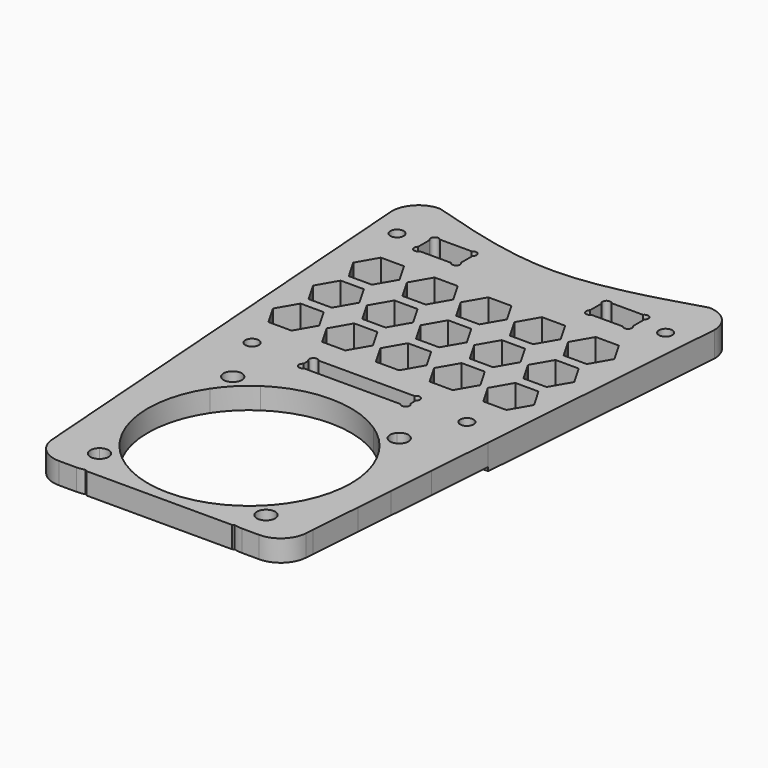
from build123d import *

# Parameters (mm, degrees)
F0_R        = 1.25
F1_DEPTH    = 4.7
F2_T1_DEPTH = 11.3905223792
F3_DEPTH    = 0.7


# Not quite as in the source:
# - a fillet or chamfer that OpenCascade refuses, or shapes differently, is made with other operations: its cross-section is extruded or revolved along the edge and cut away or added
# - a feature names something its author has since deleted; it is built from what else it names


with BuildPart() as f1:
    # F0 (on Top) → F1 (new body)
    with BuildSketch(Plane.XY):
        with BuildLine():
            ThreePointArc((-9.7202698736, -21.9205183333), (-9.7716697619, -20.7913807953), (-8.645995483, -20.8936106643))
            Line((-8.645995483, -20.8936106643), (-6.1283866754, -20.8936106643))
            Line((-6.1283866754, -20.8936106643), (-5.2063139262, -20.511675626))
            Line((-5.2063139262, -20.511675626), (0.2797301264, -20.511675626))
            Line((0.2797301264, -20.511675626), (5.7808356466, -20.511675626))
            Line((5.7808356466, -20.511675626), (6.7029083959, -20.8936106643))
            Line((6.7029083959, -20.8936106643), (9.1898135649, -20.8936106643))
            ThreePointArc((9.1898135649, -20.8936106643), (10.0314546269, -20.5883121331), (10.5658325406, -21.3066484859))
            ThreePointArc((10.5658325406, -21.3066484859), (10.4905262449, -21.6341975743), (10.2797301264, -21.8959693067))
            Line((10.2797301264, -21.8959693067), (10.2797301264, -22.3751787353))
            Line((10.2797301264, -22.3751787353), (15.9316382574, -24.7162757364))
            Line((15.9316382574, -24.7162757364), (16.8589731853, -25.6436106643))
            Line((16.8589731853, -25.6436106643), (26.7490972687, -25.6436106643))
            Line((26.7490972687, -25.6436106643), (30.2797301264, 22.5885286684))
            ThreePointArc((30.2797301264, 22.5885286684), (28.8152640324, 26.1240625744), (25.2797301264, 27.5885286684))
            add(Edge.make_bspline(
                [(-24.7202698736, 27.4813893357), (-16.3886704683, 24.9819095141), (0.2883997674, 19.9278415244), (16.944662865, 25.08800849), (25.2797301264, 27.5885286684)],
                knots=[0, 0, 0, 0, 0.4998959643, 1, 1, 1, 1], degree=3))
            ThreePointArc((-24.7202698736, 27.4813893357), (-28.2558037795, 26.0169232416), (-29.7202698736, 22.4813893357))
            Line((-29.7202698736, 22.4813893357), (-26.1974797044, -25.6436106643))
            Line((-26.1974797044, -25.6436106643), (-16.2844514649, -25.6436106643))
            Line((-16.2844514649, -25.6436106643), (-15.357116537, -24.7162757364))
            Line((-15.357116537, -24.7162757364), (-9.7202698736, -22.3814173994))
            Line((-9.7202698736, -22.3814173994), (-9.7202698736, -21.9205183333))
        make_face()
        with Locations((-19.7202698736, -22.5186106643)):
            Circle(F0_R, mode=Mode.SUBTRACT)
        Polygon((-21.9045679364, -8.5128274316), (-17.5941435837, -8.5128274316), (-15.4389314074, -12.2457644222), (-17.5941435837, -15.9787014127), (-21.9045679364, -15.9787014127), (-24.0597801128, -12.2457644222), align=None, mode=Mode.SUBTRACT)
        Polygon((-21.8574822097, 0.7808977612), (-17.547057857, 0.7808977612), (-15.3918456806, -2.9520392293), (-17.547057857, -6.6849762199), (-21.8574822097, -6.6849762199), (-24.012694386, -2.9520392293), align=None, mode=Mode.SUBTRACT)
        Polygon((-11.9045679364, -8.5128274316), (-7.5941435837, -8.5128274316), (-5.4389314074, -12.2457644222), (-7.5941435837, -15.9787014127), (-11.9045679364, -15.9787014127), (-14.0597801128, -12.2457644222), align=None, mode=Mode.SUBTRACT)
        Polygon((2.4058564163, -15.9787014127), (0.2797301264, -15.9787014127), (-1.9045679364, -15.9787014127), (-4.0597801128, -12.2457644222), (-1.9045679364, -8.5128274316), (0.2797301264, -8.5128274316), (2.4058564163, -8.5128274316), (4.5610685926, -12.2457644222), align=None, mode=Mode.SUBTRACT)
        Polygon((-11.8574822097, 0.7808977612), (-7.547057857, 0.7808977612), (-5.3918456806, -2.9520392293), (-7.547057857, -6.6849762199), (-11.8574822097, -6.6849762199), (-14.012694386, -2.9520392293), align=None, mode=Mode.SUBTRACT)
        Polygon((-21.8103964829, 10.074622954), (-17.4999721302, 10.074622954), (-15.3447599539, 6.3416859635), (-17.4999721302, 2.6087489729), (-21.8103964829, 2.6087489729), (-23.9656086593, 6.3416859635), align=None, mode=Mode.SUBTRACT)
        with Locations((-24.7202698736, 17.4813893357)):
            Circle(F0_R, mode=Mode.SUBTRACT)
        with BuildLine():
            Line((-18.6892980644, 19.8761572772), (-12.7572382877, 19.8761572772))
            ThreePointArc((-12.7572382877, 19.8761572772), (-11.9300235364, 20.0795013104), (-11.446268176, 19.3783495495))
            ThreePointArc((-11.446268176, 19.3783495495), (-11.518475663, 19.0572618523), (-11.7211943342, 18.7980006503))
            Line((-11.7211943342, 18.7980006503), (-11.7211943342, 16.1417343439))
            ThreePointArc((-11.7211943342, 16.1417343439), (-11.518475663, 15.8824731419), (-11.446268176, 15.5613854447))
            ThreePointArc((-11.446268176, 15.5613854447), (-11.9964295968, 14.8384991866), (-12.839773622, 15.1761572772))
            Line((-12.839773622, 15.1761572772), (-18.6067627301, 15.1761572772))
            ThreePointArc((-18.6067627301, 15.1761572772), (-19.7423665801, 14.9954003206), (-19.7211943342, 16.1451050294))
            Line((-19.7211943342, 16.1451050294), (-19.7211943342, 18.7946299648))
            ThreePointArc((-19.7211943342, 18.7946299648), (-19.7929027771, 19.896082772), (-18.6892980644, 19.8761572772))
        make_face(mode=Mode.SUBTRACT)
        Polygon((-11.8103964829, 10.074622954), (-7.4999721302, 10.074622954), (-5.3447599539, 6.3416859635), (-7.4999721302, 2.6087489729), (-11.8103964829, 2.6087489729), (-13.9656086593, 6.3416859635), align=None, mode=Mode.SUBTRACT)
        Polygon((8.0954320636, -8.5128274316), (12.4058564163, -8.5128274316), (14.5610685926, -12.2457644222), (12.4058564163, -15.9787014127), (8.0954320636, -15.9787014127), (5.9402198872, -12.2457644222), align=None, mode=Mode.SUBTRACT)
        Polygon((2.452942143, -6.6849762199), (0.2797301264, -6.6849762199), (-1.8574822097, -6.6849762199), (-4.012694386, -2.9520392293), (-1.8574822097, 0.7808977612), (0.2797301264, 0.7808977612), (2.452942143, 0.7808977612), (4.6081543194, -2.9520392293), align=None, mode=Mode.SUBTRACT)
        Polygon((8.1425177903, 0.7808977612), (12.452942143, 0.7808977612), (14.6081543194, -2.9520392293), (12.452942143, -6.6849762199), (8.1425177903, -6.6849762199), (5.987305614, -2.9520392293), align=None, mode=Mode.SUBTRACT)
        with Locations((20.2797301264, -22.5186106643)):
            Circle(F0_R, mode=Mode.SUBTRACT)
        Polygon((22.4058564163, -8.5128274316), (24.5610685926, -12.2457644222), (22.4058564163, -15.9787014127), (18.0954320636, -15.9787014127), (15.9402198872, -12.2457644222), (18.0954320636, -8.5128274316), align=None, mode=Mode.SUBTRACT)
        Polygon((18.1425177903, 0.7808977612), (22.452942143, 0.7808977612), (24.6081543194, -2.9520392293), (22.452942143, -6.6849762199), (18.1425177903, -6.6849762199), (15.987305614, -2.9520392293), align=None, mode=Mode.SUBTRACT)
        Polygon((2.5000278698, 2.6087489729), (0.2797301264, 2.6087489729), (-1.8103964829, 2.6087489729), (-3.9656086593, 6.3416859635), (-1.8103964829, 10.074622954), (0.2797301264, 10.074622954), (2.5000278698, 10.074622954), (4.6552400461, 6.3416859635), align=None, mode=Mode.SUBTRACT)
        Polygon((8.1896035171, 10.074622954), (12.5000278698, 10.074622954), (14.6552400461, 6.3416859635), (12.5000278698, 2.6087489729), (8.1896035171, 2.6087489729), (6.0343913407, 6.3416859635), align=None, mode=Mode.SUBTRACT)
        Polygon((18.1896035171, 10.074622954), (22.5000278698, 10.074622954), (24.6552400461, 6.3416859635), (22.5000278698, 2.6087489729), (18.1896035171, 2.6087489729), (16.0343913407, 6.3416859635), align=None, mode=Mode.SUBTRACT)
        with BuildLine():
            Line((13.3512645495, 19.8313893357), (19.2040480196, 19.8313893357))
            ThreePointArc((19.2040480196, 19.8313893357), (20.0413457449, 20.093874247), (20.5546562846, 19.3822014997))
            ThreePointArc((20.5546562846, 19.3822014997), (20.4824487976, 19.0611138025), (20.2797301264, 18.8018526005))
            Line((20.2797301264, 18.8018526005), (20.2797301264, 16.1455862941))
            ThreePointArc((20.2797301264, 16.1455862941), (20.4824487976, 15.8863250921), (20.5546562846, 15.5652373949))
            ThreePointArc((20.5546562846, 15.5652373949), (20.0323230695, 14.850627127), (19.1928753911, 15.1313893357))
            Line((19.1928753911, 15.1313893357), (13.362437178, 15.1313893357))
            ThreePointArc((13.362437178, 15.1313893357), (12.2370212083, 15.0187220626), (12.2797301264, 16.1489569796))
            Line((12.2797301264, 16.1489569796), (12.2797301264, 18.7984819149))
            ThreePointArc((12.2797301264, 18.7984819149), (12.2301480741, 19.9221748349), (13.3512645495, 19.8313893357))
        make_face(mode=Mode.SUBTRACT)
        with Locations((25.2797301264, 17.4813893357)):
            Circle(F0_R, mode=Mode.SUBTRACT)
        with BuildLine():
            Line((-9.7202698736, -23.027681977), (-9.7202698736, -22.3814173994))
            Line((-9.7202698736, -22.3814173994), (-15.357116537, -24.7162757364))
            Line((-15.357116537, -24.7162757364), (-14.737491148, -25.6436106643))
            Line((-14.737491148, -25.6436106643), (-10.6385772275, -25.6436106643))
            ThreePointArc((-10.6385772275, -25.6436106643), (-8.7305897963, -24.8128294387), (-6.7601178442, -24.1436106643))
            Line((-6.7601178442, -24.1436106643), (-8.746433961, -24.1436106643))
            ThreePointArc((-8.746433961, -24.1436106643), (-9.8878614397, -24.1568162218), (-9.7202698736, -23.027681977))
        make_face()
        with BuildLine():
            Line((0.2797301264, -24.1436106643), (-6.7601178442, -24.1436106643))
            ThreePointArc((-6.7601178442, -24.1436106643), (-8.7305897963, -24.8128294387), (-10.6385772275, -25.6436106643))
            Line((-10.6385772275, -25.6436106643), (0.2797301264, -25.6436106643))
            Line((0.2797301264, -25.6436106643), (0.2797301264, -24.1436106643))
        make_face()
        with BuildLine():
            ThreePointArc((14.4948903126, -31.5304230553), (13.4838015633, -30.71579819), (12.4261093166, -29.9626705505))
            Line((12.4261093166, -29.9626705505), (10.7936383449, -32.4058360141))
            ThreePointArc((10.7936383449, -32.4058360141), (13.6593429546, -34.757659008), (16.0111659486, -37.6233636177))
            Line((16.0111659486, -37.6233636177), (18.4543314122, -35.990892646))
            ThreePointArc((18.4543314122, -35.990892646), (17.7039036787, -34.9367639092), (16.8923918355, -33.9289059304))
            ThreePointArc((16.8923918355, -33.9289059304), (14.5774026542, -33.8454461977), (14.4948903126, -31.5304230553))
        make_face()
        with BuildLine():
            Line((14.1765166857, -27.3430007949), (12.4261093166, -29.9626705505))
            ThreePointArc((12.4261093166, -29.9626705505), (13.4838015633, -30.71579819), (14.4948903126, -31.5304230553))
            ThreePointArc((14.4948903126, -31.5304230553), (16.3737723457, -31.050778645), (17.4797301264, -32.6436106643))
            ThreePointArc((17.4797301264, -32.6436106643), (17.325939185, -33.3501781043), (16.8923918355, -33.9289059304))
            ThreePointArc((16.8923918355, -33.9289059304), (17.7039036787, -34.9367639092), (18.4543314122, -35.990892646))
            Line((18.4543314122, -35.990892646), (21.0740011678, -34.240485277))
            ThreePointArc((21.0740011678, -34.240485277), (17.9649303899, -30.4520715728), (14.1765166857, -27.3430007949))
        make_face()
        with BuildLine():
            Line((15.9316382574, -24.7162757364), (10.2797301264, -22.3751787353))
            Line((10.2797301264, -22.3751787353), (10.2797301264, -23.1251759978))
            ThreePointArc((10.2797301264, -23.1251759978), (10.5033870351, -23.3905050074), (10.5836682992, -23.7281095317))
            ThreePointArc((10.5836682992, -23.7281095317), (10.0507050937, -24.446019714), (9.209281553, -24.1436106643))
            Line((9.209281553, -24.1436106643), (7.3346395646, -24.1436106643))
            ThreePointArc((7.3346395646, -24.1436106643), (9.3051115167, -24.8128294387), (11.2130989479, -25.6436106643))
            Line((11.2130989479, -25.6436106643), (15.3120128685, -25.6436106643))
            Line((15.3120128685, -25.6436106643), (15.9316382574, -24.7162757364))
        make_face()
        Polygon((16.8589731853, -25.6436106643), (15.9316382574, -24.7162757364), (15.3120128685, -25.6436106643), align=None)
        with BuildLine():
            Line((23.7007262262, -32.4853637052), (16.8589731853, -25.6436106643))
            Line((16.8589731853, -25.6436106643), (15.3120128685, -25.6436106643))
            Line((15.3120128685, -25.6436106643), (14.1765166857, -27.3430007949))
            ThreePointArc((14.1765166857, -27.3430007949), (17.9649303899, -30.4520715728), (21.0740011678, -34.240485277))
            Line((21.0740011678, -34.240485277), (23.7007262262, -32.4853637052))
        make_face()
        with BuildLine():
            Line((-14.737491148, -25.6436106643), (-16.2844514649, -25.6436106643))
            Line((-16.2844514649, -25.6436106643), (-23.1262045058, -32.4853637052))
            Line((-23.1262045058, -32.4853637052), (-20.4994794474, -34.240485277))
            ThreePointArc((-20.4994794474, -34.240485277), (-17.3904086695, -30.4520715728), (-13.6019949653, -27.3430007949))
            Line((-13.6019949653, -27.3430007949), (-14.737491148, -25.6436106643))
        make_face()
        Polygon((-14.737491148, -25.6436106643), (-15.357116537, -24.7162757364), (-16.2844514649, -25.6436106643), align=None)
        with BuildLine():
            Line((-11.8515875962, -29.9626705505), (-13.6019949653, -27.3430007949))
            ThreePointArc((-13.6019949653, -27.3430007949), (-17.3904086695, -30.4520715728), (-20.4994794474, -34.240485277))
            Line((-20.4994794474, -34.240485277), (-17.8798096918, -35.990892646))
            ThreePointArc((-17.8798096918, -35.990892646), (-17.1323460944, -34.9406779122), (-16.3242505384, -33.9363699968))
            ThreePointArc((-16.3242505384, -33.9363699968), (-16.42318112, -31.4423594278), (-13.9290363114, -31.5378458214))
            ThreePointArc((-13.9290363114, -31.5378458214), (-12.9138269568, -30.7192449942), (-11.8515875962, -29.9626705505))
        make_face()
        with BuildLine():
            Line((-10.2191166245, -32.4058360141), (-11.8515875962, -29.9626705505))
            ThreePointArc((-11.8515875962, -29.9626705505), (-12.9138269568, -30.7192449942), (-13.9290363114, -31.5378458214))
            ThreePointArc((-13.9290363114, -31.5378458214), (-13.6257327847, -32.0541605204), (-13.5202698736, -32.6436106643))
            ThreePointArc((-13.5202698736, -32.6436106643), (-14.5084999424, -34.1874317566), (-16.3242505384, -33.9363699968))
            ThreePointArc((-16.3242505384, -33.9363699968), (-17.1323460944, -34.9406779122), (-17.8798096918, -35.990892646))
            Line((-17.8798096918, -35.990892646), (-15.4366442282, -37.6233636177))
            ThreePointArc((-15.4366442282, -37.6233636177), (-13.0848212342, -34.757659008), (-10.2191166245, -32.4058360141))
        make_face()
        with BuildLine():
            ThreePointArc((-16.3104778398, -62.3392155591), (-17.1259485967, -61.3272496059), (-17.8798096918, -60.2685895589))
            Line((-17.8798096918, -60.2685895589), (-20.4994794474, -62.0189969279))
            ThreePointArc((-20.4994794474, -62.0189969279), (-17.3904086695, -65.8074106321), (-13.6019949653, -68.91648141))
            Line((-13.6019949653, -68.91648141), (-11.8515875962, -66.2968116544))
            ThreePointArc((-11.8515875962, -66.2968116544), (-12.9066892002, -65.5456469386), (-13.9154293371, -64.7332854665))
            ThreePointArc((-13.9154293371, -64.7332854665), (-16.4221057464, -64.8459377973), (-16.3104778398, -62.3392155591))
        make_face()
        with BuildLine():
            Line((-15.4366442282, -58.6361185872), (-17.8798096918, -60.2685895589))
            ThreePointArc((-17.8798096918, -60.2685895589), (-17.1259485967, -61.3272496059), (-16.3104778398, -62.3392155591))
            ThreePointArc((-16.3104778398, -62.3392155591), (-14.5003231889, -62.1035857387), (-13.5202698736, -63.6436106643))
            ThreePointArc((-13.5202698736, -63.6436106643), (-13.6221101644, -64.2231669981), (-13.9154293371, -64.7332854665))
            ThreePointArc((-13.9154293371, -64.7332854665), (-12.9066892002, -65.5456469386), (-11.8515875962, -66.2968116544))
            Line((-11.8515875962, -66.2968116544), (-10.2191166245, -63.8536461909))
            ThreePointArc((-10.2191166245, -63.8536461909), (-13.0848212342, -61.5018231969), (-15.4366442282, -58.6361185872))
        make_face()
        with BuildLine():
            ThreePointArc((-13.6019949653, -68.91648141), (-17.3904086695, -65.8074106321), (-20.4994794474, -62.0189969279))
            Line((-20.4994794474, -62.0189969279), (-23.1262045058, -63.7741184997))
            Line((-23.1262045058, -63.7741184997), (-17.7567123412, -69.1436106643))
            Line((-17.7567123412, -69.1436106643), (-13.753757881, -69.1436106643))
            Line((-13.753757881, -69.1436106643), (-13.6019949653, -68.91648141))
        make_face()
        with BuildLine():
            Line((-23.1262045058, -63.7741184997), (-23.4664180794, -62.9527702762))
            Line((-23.4664180794, -62.9527702762), (-23.352527251, -64.5086381695))
            ThreePointArc((-23.352527251, -64.5086381695), (-21.7699011758, -67.8059280677), (-18.3658695606, -69.1436106643))
            Line((-18.3658695606, -69.1436106643), (-17.7567123412, -69.1436106643))
            Line((-17.7567123412, -69.1436106643), (-23.1262045058, -63.7741184997))
        make_face()
        with BuildLine():
            ThreePointArc((16.0111659486, -58.6361185872), (13.6593429546, -61.5018231969), (10.7936383449, -63.8536461909))
            Line((10.7936383449, -63.8536461909), (12.4261093166, -66.2968116544))
            ThreePointArc((12.4261093166, -66.2968116544), (13.4766140098, -65.5491285137), (14.4811849778, -64.7407799753))
            ThreePointArc((14.4811849778, -64.7407799753), (14.5784785504, -62.4406997569), (16.8786908795, -62.3465812648))
            ThreePointArc((16.8786908795, -62.3465812648), (17.697540952, -61.3311138119), (18.4543314122, -60.2685895589))
            Line((18.4543314122, -60.2685895589), (16.0111659486, -58.6361185872))
        make_face()
        with BuildLine():
            ThreePointArc((14.1765166857, -68.91648141), (17.9649303899, -65.8074106321), (21.0740011678, -62.0189969279))
            Line((21.0740011678, -62.0189969279), (18.4543314122, -60.2685895589))
            ThreePointArc((18.4543314122, -60.2685895589), (17.697540952, -61.3311138119), (16.8786908795, -62.3465812648))
            ThreePointArc((16.8786908795, -62.3465812648), (17.3221686633, -62.9288496134), (17.4797301264, -63.6436106643))
            ThreePointArc((17.4797301264, -63.6436106643), (16.3638847495, -65.2400953577), (14.4811849778, -64.7407799753))
            ThreePointArc((14.4811849778, -64.7407799753), (13.4766140098, -65.5491285137), (12.4261093166, -66.2968116544))
            Line((12.4261093166, -66.2968116544), (14.1765166857, -68.91648141))
        make_face()
        with BuildLine():
            Line((23.7007262262, -63.7741184997), (21.0740011678, -62.0189969279))
            ThreePointArc((21.0740011678, -62.0189969279), (17.9649303899, -65.8074106321), (14.1765166857, -68.91648141))
            Line((14.1765166857, -68.91648141), (14.3282796014, -69.1436106643))
            Line((14.3282796014, -69.1436106643), (18.3312340616, -69.1436106643))
            Line((18.3312340616, -69.1436106643), (23.7007262262, -63.7741184997))
        make_face()
        with BuildLine():
            Line((23.9041448152, -64.5086381695), (24.0131191018, -63.0199353826))
            Line((24.0131191018, -63.0199353826), (23.7007262262, -63.7741184997))
            Line((23.7007262262, -63.7741184997), (18.3312340616, -69.1436106643))
            Line((18.3312340616, -69.1436106643), (18.9174871249, -69.1436106643))
            ThreePointArc((18.9174871249, -69.1436106643), (22.3215187401, -67.8059280677), (23.9041448152, -64.5086381695))
        make_face()
        with BuildLine():
            Line((-10.6385772275, -25.6436106643), (-14.737491148, -25.6436106643))
            Line((-14.737491148, -25.6436106643), (-13.6019949653, -27.3430007949))
            ThreePointArc((-13.6019949653, -27.3430007949), (-12.1493465222, -26.4426297961), (-10.6385772275, -25.6436106643))
        make_face()
        with BuildLine():
            Line((7.3346395646, -24.1436106643), (0.2797301264, -24.1436106643))
            Line((0.2797301264, -24.1436106643), (0.2797301264, -25.6436106643))
            Line((0.2797301264, -25.6436106643), (11.2130989479, -25.6436106643))
            ThreePointArc((11.2130989479, -25.6436106643), (9.3051115167, -24.8128294387), (7.3346395646, -24.1436106643))
        make_face()
        with BuildLine():
            Line((14.1765166857, -27.3430007949), (15.3120128685, -25.6436106643))
            Line((15.3120128685, -25.6436106643), (11.2130989479, -25.6436106643))
            ThreePointArc((11.2130989479, -25.6436106643), (12.7238682426, -26.4426297961), (14.1765166857, -27.3430007949))
        make_face()
        with BuildLine():
            ThreePointArc((-10.6385772275, -25.6436106643), (-12.1493465222, -26.4426297961), (-13.6019949653, -27.3430007949))
            Line((-13.6019949653, -27.3430007949), (-11.8515875962, -29.9626705505))
            ThreePointArc((-11.8515875962, -29.9626705505), (0.2872608602, -26.2803911284), (12.4261093166, -29.9626705505))
            Line((12.4261093166, -29.9626705505), (14.1765166857, -27.3430007949))
            ThreePointArc((14.1765166857, -27.3430007949), (12.7238682426, -26.4426297961), (11.2130989479, -25.6436106643))
            Line((11.2130989479, -25.6436106643), (0.2797301264, -25.6436106643))
            Line((0.2797301264, -25.6436106643), (-10.6385772275, -25.6436106643))
        make_face()
        Polygon((-5.2063139262, -20.511675626), (-6.1283866754, -20.8936106643), (0.2797301264, -20.8936106643), (0.2797301264, -20.511675626), align=None)
        Polygon((0.2797301264, -20.511675626), (0.2797301264, -20.8936106643), (6.7029083959, -20.8936106643), (5.7808356466, -20.511675626), align=None)
        Polygon((-23.1262045058, -32.4853637052), (-16.2844514649, -25.6436106643), (-26.1974797044, -25.6436106643), (-25.3106220547, -37.7590141775), align=None)
        with BuildLine():
            ThreePointArc((12.4261093166, -29.9626705505), (0.2872608602, -26.2803911284), (-11.8515875962, -29.9626705505))
            Line((-11.8515875962, -29.9626705505), (-10.2191166245, -32.4058360141))
            ThreePointArc((-10.2191166245, -32.4058360141), (0.2872608602, -29.2187612473), (10.7936383449, -32.4058360141))
            Line((10.7936383449, -32.4058360141), (12.4261093166, -29.9626705505))
        make_face()
        with BuildLine():
            Line((-20.4994794474, -34.240485277), (-23.1262045058, -32.4853637052))
            Line((-23.1262045058, -32.4853637052), (-25.3106220547, -37.7590141775))
            Line((-25.3106220547, -37.7590141775), (-24.6647780638, -46.5819189115))
            ThreePointArc((-24.6647780638, -46.5819189115), (-23.4000084513, -40.1351634049), (-20.4994794474, -34.240485277))
        make_face()
        with BuildLine():
            Line((-17.8798096918, -35.990892646), (-20.4994794474, -34.240485277))
            ThreePointArc((-20.4994794474, -34.240485277), (-23.4000084513, -40.1351634049), (-24.6647780638, -46.5819189115))
            Line((-24.6647780638, -46.5819189115), (-24.1734031516, -53.2946143923))
            ThreePointArc((-24.1734031516, -53.2946143923), (-22.7531517244, -57.8322865382), (-20.4994794474, -62.0189969279))
            Line((-20.4994794474, -62.0189969279), (-17.8798096918, -60.2685895589))
            ThreePointArc((-17.8798096918, -60.2685895589), (-21.5620891139, -48.1297411025), (-17.8798096918, -35.990892646))
        make_face()
        with BuildLine():
            Line((-15.4366442282, -37.6233636177), (-17.8798096918, -35.990892646))
            ThreePointArc((-17.8798096918, -35.990892646), (-21.5620891139, -48.1297411025), (-17.8798096918, -60.2685895589))
            Line((-17.8798096918, -60.2685895589), (-15.4366442282, -58.6361185872))
            ThreePointArc((-15.4366442282, -58.6361185872), (-18.6237189949, -48.1297411025), (-15.4366442282, -37.6233636177))
        make_face()
        with BuildLine():
            ThreePointArc((-20.4994794474, -62.0189969279), (-22.7531517244, -57.8322865382), (-24.1734031516, -53.2946143923))
            Line((-24.1734031516, -53.2946143923), (-23.4664180794, -62.9527702762))
            Line((-23.4664180794, -62.9527702762), (-23.1262045058, -63.7741184997))
            Line((-23.1262045058, -63.7741184997), (-20.4994794474, -62.0189969279))
        make_face()
        Polygon((26.7490972687, -25.6436106643), (16.8589731853, -25.6436106643), (23.7007262262, -32.4853637052), (25.8656794093, -37.7120230417), align=None)
        with BuildLine():
            Line((25.8656794093, -37.7120230417), (23.7007262262, -32.4853637052))
            Line((23.7007262262, -32.4853637052), (21.0740011678, -34.240485277))
            ThreePointArc((21.0740011678, -34.240485277), (23.9479133476, -40.0567290331), (25.2284958887, -46.4166166896))
            Line((25.2284958887, -46.4166166896), (25.8656794093, -37.7120230417))
        make_face()
        with BuildLine():
            ThreePointArc((25.2284958887, -46.4166166896), (23.9479133476, -40.0567290331), (21.0740011678, -34.240485277))
            Line((21.0740011678, -34.240485277), (18.4543314122, -35.990892646))
            ThreePointArc((18.4543314122, -35.990892646), (21.1957851599, -41.787209597), (22.1366108343, -48.1297411025))
            ThreePointArc((22.1366108343, -48.1297411025), (21.1957851599, -54.4722726079), (18.4543314122, -60.2685895589))
            Line((18.4543314122, -60.2685895589), (21.0740011678, -62.0189969279))
            ThreePointArc((21.0740011678, -62.0189969279), (23.295401506, -57.9085684362), (24.7131646046, -53.4565812794))
            Line((24.7131646046, -53.4565812794), (25.2284958887, -46.4166166896))
        make_face()
        with BuildLine():
            Line((18.4543314122, -35.990892646), (16.0111659486, -37.6233636177))
            ThreePointArc((16.0111659486, -37.6233636177), (18.3839402718, -42.6401734186), (19.1982407153, -48.1297411025))
            ThreePointArc((19.1982407153, -48.1297411025), (18.3839402718, -53.6193087863), (16.0111659486, -58.6361185872))
            Line((16.0111659486, -58.6361185872), (18.4543314122, -60.2685895589))
            ThreePointArc((18.4543314122, -60.2685895589), (21.1957851599, -54.4722726079), (22.1366108343, -48.1297411025))
            ThreePointArc((22.1366108343, -48.1297411025), (21.1957851599, -41.787209597), (18.4543314122, -35.990892646))
        make_face()
        with BuildLine():
            ThreePointArc((10.7936383449, -63.8536461909), (0.2872608602, -67.0407209576), (-10.2191166245, -63.8536461909))
            Line((-10.2191166245, -63.8536461909), (-11.8515875962, -66.2968116544))
            ThreePointArc((-11.8515875962, -66.2968116544), (-8.8854072743, -67.9604307925), (-5.6970001908, -69.1436106643))
            Line((-5.6970001908, -69.1436106643), (6.2715219113, -69.1436106643))
            ThreePointArc((6.2715219113, -69.1436106643), (9.4599289947, -67.9604307925), (12.4261093166, -66.2968116544))
            Line((12.4261093166, -66.2968116544), (10.7936383449, -63.8536461909))
        make_face()
        with BuildLine():
            Line((-11.8515875962, -66.2968116544), (-13.6019949653, -68.91648141))
            ThreePointArc((-13.6019949653, -68.91648141), (-13.4294190849, -69.0307624001), (-13.2559029518, -69.1436106643))
            Line((-13.2559029518, -69.1436106643), (-5.6970001908, -69.1436106643))
            ThreePointArc((-5.6970001908, -69.1436106643), (-8.8854072743, -67.9604307925), (-11.8515875962, -66.2968116544))
        make_face()
        with BuildLine():
            Line((14.1765166857, -68.91648141), (12.4261093166, -66.2968116544))
            ThreePointArc((12.4261093166, -66.2968116544), (9.4599289947, -67.9604307925), (6.2715219113, -69.1436106643))
            Line((6.2715219113, -69.1436106643), (13.8304246722, -69.1436106643))
            ThreePointArc((13.8304246722, -69.1436106643), (14.0039408053, -69.0307624001), (14.1765166857, -68.91648141))
        make_face()
        with BuildLine():
            Line((24.0131191018, -63.0199353826), (24.7131646046, -53.4565812794))
            ThreePointArc((24.7131646046, -53.4565812794), (23.295401506, -57.9085684362), (21.0740011678, -62.0189969279))
            Line((21.0740011678, -62.0189969279), (23.7007262262, -63.7741184997))
            Line((23.7007262262, -63.7741184997), (24.0131191018, -63.0199353826))
        make_face()
    extrude(amount=F1_DEPTH)

    # F2: fillet of radius 5 on 2 edges, made by hand

    # F2_s2 → F2_t1 (cut)
    with BuildSketch(Plane.XY.offset(-3.3452611896)):
        with BuildLine():
            ThreePointArc((14.1765166857, -68.91648141), (14.9128436765, -69.0865022132), (15.6663840773, -69.1436106643))
            Line((15.6663840773, -69.1436106643), (14.3282796014, -69.1436106643))
            Line((14.3282796014, -69.1436106643), (14.1765166857, -68.91648141))
        make_face()
        with BuildLine():
            ThreePointArc((-15.0918623569, -69.1436106643), (-14.3383219561, -69.0865022132), (-13.6019949653, -68.91648141))
            Line((-13.6019949653, -68.91648141), (-13.753757881, -69.1436106643))
            Line((-13.753757881, -69.1436106643), (-15.0918623569, -69.1436106643))
        make_face()
    extrude(amount=F2_T1_DEPTH, mode=Mode.SUBTRACT)

    # F0 (on Top) → F3 (cut)
    with BuildSketch(Plane.XY):
        with BuildLine():
            Line((-14.737491148, -25.6436106643), (-16.2844514649, -25.6436106643))
            Line((-16.2844514649, -25.6436106643), (-23.1262045058, -32.4853637052))
            Line((-23.1262045058, -32.4853637052), (-20.4994794474, -34.240485277))
            ThreePointArc((-20.4994794474, -34.240485277), (-17.3904086695, -30.4520715728), (-13.6019949653, -27.3430007949))
            Line((-13.6019949653, -27.3430007949), (-14.737491148, -25.6436106643))
        make_face()
        with BuildLine():
            Line((-10.6385772275, -25.6436106643), (-14.737491148, -25.6436106643))
            Line((-14.737491148, -25.6436106643), (-13.6019949653, -27.3430007949))
            ThreePointArc((-13.6019949653, -27.3430007949), (-12.1493465222, -26.4426297961), (-10.6385772275, -25.6436106643))
        make_face()
        with BuildLine():
            ThreePointArc((-10.6385772275, -25.6436106643), (-12.1493465222, -26.4426297961), (-13.6019949653, -27.3430007949))
            Line((-13.6019949653, -27.3430007949), (-11.8515875962, -29.9626705505))
            ThreePointArc((-11.8515875962, -29.9626705505), (0.2872608602, -26.2803911284), (12.4261093166, -29.9626705505))
            Line((12.4261093166, -29.9626705505), (14.1765166857, -27.3430007949))
            ThreePointArc((14.1765166857, -27.3430007949), (12.7238682426, -26.4426297961), (11.2130989479, -25.6436106643))
            Line((11.2130989479, -25.6436106643), (0.2797301264, -25.6436106643))
            Line((0.2797301264, -25.6436106643), (-10.6385772275, -25.6436106643))
        make_face()
        with BuildLine():
            Line((-11.8515875962, -29.9626705505), (-13.6019949653, -27.3430007949))
            ThreePointArc((-13.6019949653, -27.3430007949), (-17.3904086695, -30.4520715728), (-20.4994794474, -34.240485277))
            Line((-20.4994794474, -34.240485277), (-17.8798096918, -35.990892646))
            ThreePointArc((-17.8798096918, -35.990892646), (-17.1323460944, -34.9406779122), (-16.3242505384, -33.9363699968))
            ThreePointArc((-16.3242505384, -33.9363699968), (-16.42318112, -31.4423594278), (-13.9290363114, -31.5378458214))
            ThreePointArc((-13.9290363114, -31.5378458214), (-12.9138269568, -30.7192449942), (-11.8515875962, -29.9626705505))
        make_face()
        with BuildLine():
            Line((-10.2191166245, -32.4058360141), (-11.8515875962, -29.9626705505))
            ThreePointArc((-11.8515875962, -29.9626705505), (-12.9138269568, -30.7192449942), (-13.9290363114, -31.5378458214))
            ThreePointArc((-13.9290363114, -31.5378458214), (-13.6257327847, -32.0541605204), (-13.5202698736, -32.6436106643))
            ThreePointArc((-13.5202698736, -32.6436106643), (-14.5084999424, -34.1874317566), (-16.3242505384, -33.9363699968))
            ThreePointArc((-16.3242505384, -33.9363699968), (-17.1323460944, -34.9406779122), (-17.8798096918, -35.990892646))
            Line((-17.8798096918, -35.990892646), (-15.4366442282, -37.6233636177))
            ThreePointArc((-15.4366442282, -37.6233636177), (-13.0848212342, -34.757659008), (-10.2191166245, -32.4058360141))
        make_face()
        with BuildLine():
            Line((14.1765166857, -27.3430007949), (15.3120128685, -25.6436106643))
            Line((15.3120128685, -25.6436106643), (11.2130989479, -25.6436106643))
            ThreePointArc((11.2130989479, -25.6436106643), (12.7238682426, -26.4426297961), (14.1765166857, -27.3430007949))
        make_face()
        with BuildLine():
            Line((23.7007262262, -32.4853637052), (16.8589731853, -25.6436106643))
            Line((16.8589731853, -25.6436106643), (15.3120128685, -25.6436106643))
            Line((15.3120128685, -25.6436106643), (14.1765166857, -27.3430007949))
            ThreePointArc((14.1765166857, -27.3430007949), (17.9649303899, -30.4520715728), (21.0740011678, -34.240485277))
            Line((21.0740011678, -34.240485277), (23.7007262262, -32.4853637052))
        make_face()
        with BuildLine():
            ThreePointArc((14.4948903126, -31.5304230553), (13.4838015633, -30.71579819), (12.4261093166, -29.9626705505))
            Line((12.4261093166, -29.9626705505), (10.7936383449, -32.4058360141))
            ThreePointArc((10.7936383449, -32.4058360141), (13.6593429546, -34.757659008), (16.0111659486, -37.6233636177))
            Line((16.0111659486, -37.6233636177), (18.4543314122, -35.990892646))
            ThreePointArc((18.4543314122, -35.990892646), (17.7039036787, -34.9367639092), (16.8923918355, -33.9289059304))
            ThreePointArc((16.8923918355, -33.9289059304), (14.5774026542, -33.8454461977), (14.4948903126, -31.5304230553))
        make_face()
        with BuildLine():
            Line((14.1765166857, -27.3430007949), (12.4261093166, -29.9626705505))
            ThreePointArc((12.4261093166, -29.9626705505), (13.4838015633, -30.71579819), (14.4948903126, -31.5304230553))
            ThreePointArc((14.4948903126, -31.5304230553), (16.3737723457, -31.050778645), (17.4797301264, -32.6436106643))
            ThreePointArc((17.4797301264, -32.6436106643), (17.325939185, -33.3501781043), (16.8923918355, -33.9289059304))
            ThreePointArc((16.8923918355, -33.9289059304), (17.7039036787, -34.9367639092), (18.4543314122, -35.990892646))
            Line((18.4543314122, -35.990892646), (21.0740011678, -34.240485277))
            ThreePointArc((21.0740011678, -34.240485277), (17.9649303899, -30.4520715728), (14.1765166857, -27.3430007949))
        make_face()
        with BuildLine():
            Line((23.7007262262, -63.7741184997), (21.0740011678, -62.0189969279))
            ThreePointArc((21.0740011678, -62.0189969279), (17.9649303899, -65.8074106321), (14.1765166857, -68.91648141))
            Line((14.1765166857, -68.91648141), (14.3282796014, -69.1436106643))
            Line((14.3282796014, -69.1436106643), (18.3312340616, -69.1436106643))
            Line((18.3312340616, -69.1436106643), (23.7007262262, -63.7741184997))
        make_face()
        with BuildLine():
            ThreePointArc((16.0111659486, -58.6361185872), (13.6593429546, -61.5018231969), (10.7936383449, -63.8536461909))
            Line((10.7936383449, -63.8536461909), (12.4261093166, -66.2968116544))
            ThreePointArc((12.4261093166, -66.2968116544), (13.4766140098, -65.5491285137), (14.4811849778, -64.7407799753))
            ThreePointArc((14.4811849778, -64.7407799753), (14.5784785504, -62.4406997569), (16.8786908795, -62.3465812648))
            ThreePointArc((16.8786908795, -62.3465812648), (17.697540952, -61.3311138119), (18.4543314122, -60.2685895589))
            Line((18.4543314122, -60.2685895589), (16.0111659486, -58.6361185872))
        make_face()
        with BuildLine():
            ThreePointArc((14.1765166857, -68.91648141), (17.9649303899, -65.8074106321), (21.0740011678, -62.0189969279))
            Line((21.0740011678, -62.0189969279), (18.4543314122, -60.2685895589))
            ThreePointArc((18.4543314122, -60.2685895589), (17.697540952, -61.3311138119), (16.8786908795, -62.3465812648))
            ThreePointArc((16.8786908795, -62.3465812648), (17.3221686633, -62.9288496134), (17.4797301264, -63.6436106643))
            ThreePointArc((17.4797301264, -63.6436106643), (16.3638847495, -65.2400953577), (14.4811849778, -64.7407799753))
            ThreePointArc((14.4811849778, -64.7407799753), (13.4766140098, -65.5491285137), (12.4261093166, -66.2968116544))
            Line((12.4261093166, -66.2968116544), (14.1765166857, -68.91648141))
        make_face()
        with BuildLine():
            Line((23.9041448152, -64.5086381695), (24.0131191018, -63.0199353826))
            Line((24.0131191018, -63.0199353826), (23.7007262262, -63.7741184997))
            Line((23.7007262262, -63.7741184997), (18.3312340616, -69.1436106643))
            Line((18.3312340616, -69.1436106643), (18.9174871249, -69.1436106643))
            ThreePointArc((18.9174871249, -69.1436106643), (22.3215187401, -67.8059280677), (23.9041448152, -64.5086381695))
        make_face()
        with BuildLine():
            Line((-15.4366442282, -58.6361185872), (-17.8798096918, -60.2685895589))
            ThreePointArc((-17.8798096918, -60.2685895589), (-17.1259485967, -61.3272496059), (-16.3104778398, -62.3392155591))
            ThreePointArc((-16.3104778398, -62.3392155591), (-14.5003231889, -62.1035857387), (-13.5202698736, -63.6436106643))
            ThreePointArc((-13.5202698736, -63.6436106643), (-13.6221101644, -64.2231669981), (-13.9154293371, -64.7332854665))
            ThreePointArc((-13.9154293371, -64.7332854665), (-12.9066892002, -65.5456469386), (-11.8515875962, -66.2968116544))
            Line((-11.8515875962, -66.2968116544), (-10.2191166245, -63.8536461909))
            ThreePointArc((-10.2191166245, -63.8536461909), (-13.0848212342, -61.5018231969), (-15.4366442282, -58.6361185872))
        make_face()
        with BuildLine():
            ThreePointArc((-16.3104778398, -62.3392155591), (-17.1259485967, -61.3272496059), (-17.8798096918, -60.2685895589))
            Line((-17.8798096918, -60.2685895589), (-20.4994794474, -62.0189969279))
            ThreePointArc((-20.4994794474, -62.0189969279), (-17.3904086695, -65.8074106321), (-13.6019949653, -68.91648141))
            Line((-13.6019949653, -68.91648141), (-11.8515875962, -66.2968116544))
            ThreePointArc((-11.8515875962, -66.2968116544), (-12.9066892002, -65.5456469386), (-13.9154293371, -64.7332854665))
            ThreePointArc((-13.9154293371, -64.7332854665), (-16.4221057464, -64.8459377973), (-16.3104778398, -62.3392155591))
        make_face()
        with BuildLine():
            ThreePointArc((-13.6019949653, -68.91648141), (-17.3904086695, -65.8074106321), (-20.4994794474, -62.0189969279))
            Line((-20.4994794474, -62.0189969279), (-23.1262045058, -63.7741184997))
            Line((-23.1262045058, -63.7741184997), (-17.7567123412, -69.1436106643))
            Line((-17.7567123412, -69.1436106643), (-13.753757881, -69.1436106643))
            Line((-13.753757881, -69.1436106643), (-13.6019949653, -68.91648141))
        make_face()
        with BuildLine():
            Line((-23.1262045058, -63.7741184997), (-23.4664180794, -62.9527702762))
            Line((-23.4664180794, -62.9527702762), (-23.352527251, -64.5086381695))
            ThreePointArc((-23.352527251, -64.5086381695), (-21.7699011758, -67.8059280677), (-18.3658695606, -69.1436106643))
            Line((-18.3658695606, -69.1436106643), (-17.7567123412, -69.1436106643))
            Line((-17.7567123412, -69.1436106643), (-23.1262045058, -63.7741184997))
        make_face()
        Polygon((-23.1262045058, -32.4853637052), (-16.2844514649, -25.6436106643), (-26.1974797044, -25.6436106643), (-25.3106220547, -37.7590141775), align=None)
        with BuildLine():
            ThreePointArc((12.4261093166, -29.9626705505), (0.2872608602, -26.2803911284), (-11.8515875962, -29.9626705505))
            Line((-11.8515875962, -29.9626705505), (-10.2191166245, -32.4058360141))
            ThreePointArc((-10.2191166245, -32.4058360141), (0.2872608602, -29.2187612473), (10.7936383449, -32.4058360141))
            Line((10.7936383449, -32.4058360141), (12.4261093166, -29.9626705505))
        make_face()
        Polygon((26.7490972687, -25.6436106643), (16.8589731853, -25.6436106643), (23.7007262262, -32.4853637052), (25.8656794093, -37.7120230417), align=None)
        with BuildLine():
            Line((25.8656794093, -37.7120230417), (23.7007262262, -32.4853637052))
            Line((23.7007262262, -32.4853637052), (21.0740011678, -34.240485277))
            ThreePointArc((21.0740011678, -34.240485277), (23.9479133476, -40.0567290331), (25.2284958887, -46.4166166896))
            Line((25.2284958887, -46.4166166896), (25.8656794093, -37.7120230417))
        make_face()
        with BuildLine():
            ThreePointArc((25.2284958887, -46.4166166896), (23.9479133476, -40.0567290331), (21.0740011678, -34.240485277))
            Line((21.0740011678, -34.240485277), (18.4543314122, -35.990892646))
            ThreePointArc((18.4543314122, -35.990892646), (21.1957851599, -41.787209597), (22.1366108343, -48.1297411025))
            ThreePointArc((22.1366108343, -48.1297411025), (21.1957851599, -54.4722726079), (18.4543314122, -60.2685895589))
            Line((18.4543314122, -60.2685895589), (21.0740011678, -62.0189969279))
            ThreePointArc((21.0740011678, -62.0189969279), (23.295401506, -57.9085684362), (24.7131646046, -53.4565812794))
            Line((24.7131646046, -53.4565812794), (25.2284958887, -46.4166166896))
        make_face()
        with BuildLine():
            Line((18.4543314122, -35.990892646), (16.0111659486, -37.6233636177))
            ThreePointArc((16.0111659486, -37.6233636177), (18.3839402718, -42.6401734186), (19.1982407153, -48.1297411025))
            ThreePointArc((19.1982407153, -48.1297411025), (18.3839402718, -53.6193087863), (16.0111659486, -58.6361185872))
            Line((16.0111659486, -58.6361185872), (18.4543314122, -60.2685895589))
            ThreePointArc((18.4543314122, -60.2685895589), (21.1957851599, -54.4722726079), (22.1366108343, -48.1297411025))
            ThreePointArc((22.1366108343, -48.1297411025), (21.1957851599, -41.787209597), (18.4543314122, -35.990892646))
        make_face()
        with BuildLine():
            Line((24.0131191018, -63.0199353826), (24.7131646046, -53.4565812794))
            ThreePointArc((24.7131646046, -53.4565812794), (23.295401506, -57.9085684362), (21.0740011678, -62.0189969279))
            Line((21.0740011678, -62.0189969279), (23.7007262262, -63.7741184997))
            Line((23.7007262262, -63.7741184997), (24.0131191018, -63.0199353826))
        make_face()
        with BuildLine():
            Line((14.1765166857, -68.91648141), (12.4261093166, -66.2968116544))
            ThreePointArc((12.4261093166, -66.2968116544), (9.4599289947, -67.9604307925), (6.2715219113, -69.1436106643))
            Line((6.2715219113, -69.1436106643), (13.8304246722, -69.1436106643))
            ThreePointArc((13.8304246722, -69.1436106643), (14.0039408053, -69.0307624001), (14.1765166857, -68.91648141))
        make_face()
        with BuildLine():
            ThreePointArc((10.7936383449, -63.8536461909), (0.2872608602, -67.0407209576), (-10.2191166245, -63.8536461909))
            Line((-10.2191166245, -63.8536461909), (-11.8515875962, -66.2968116544))
            ThreePointArc((-11.8515875962, -66.2968116544), (-8.8854072743, -67.9604307925), (-5.6970001908, -69.1436106643))
            Line((-5.6970001908, -69.1436106643), (6.2715219113, -69.1436106643))
            ThreePointArc((6.2715219113, -69.1436106643), (9.4599289947, -67.9604307925), (12.4261093166, -66.2968116544))
            Line((12.4261093166, -66.2968116544), (10.7936383449, -63.8536461909))
        make_face()
        with BuildLine():
            Line((-11.8515875962, -66.2968116544), (-13.6019949653, -68.91648141))
            ThreePointArc((-13.6019949653, -68.91648141), (-13.4294190849, -69.0307624001), (-13.2559029518, -69.1436106643))
            Line((-13.2559029518, -69.1436106643), (-5.6970001908, -69.1436106643))
            ThreePointArc((-5.6970001908, -69.1436106643), (-8.8854072743, -67.9604307925), (-11.8515875962, -66.2968116544))
        make_face()
        with BuildLine():
            Line((-15.4366442282, -37.6233636177), (-17.8798096918, -35.990892646))
            ThreePointArc((-17.8798096918, -35.990892646), (-21.5620891139, -48.1297411025), (-17.8798096918, -60.2685895589))
            Line((-17.8798096918, -60.2685895589), (-15.4366442282, -58.6361185872))
            ThreePointArc((-15.4366442282, -58.6361185872), (-18.6237189949, -48.1297411025), (-15.4366442282, -37.6233636177))
        make_face()
        with BuildLine():
            Line((-17.8798096918, -35.990892646), (-20.4994794474, -34.240485277))
            ThreePointArc((-20.4994794474, -34.240485277), (-23.4000084513, -40.1351634049), (-24.6647780638, -46.5819189115))
            Line((-24.6647780638, -46.5819189115), (-24.1734031516, -53.2946143923))
            ThreePointArc((-24.1734031516, -53.2946143923), (-22.7531517244, -57.8322865382), (-20.4994794474, -62.0189969279))
            Line((-20.4994794474, -62.0189969279), (-17.8798096918, -60.2685895589))
            ThreePointArc((-17.8798096918, -60.2685895589), (-21.5620891139, -48.1297411025), (-17.8798096918, -35.990892646))
        make_face()
        with BuildLine():
            ThreePointArc((-20.4994794474, -62.0189969279), (-22.7531517244, -57.8322865382), (-24.1734031516, -53.2946143923))
            Line((-24.1734031516, -53.2946143923), (-23.4664180794, -62.9527702762))
            Line((-23.4664180794, -62.9527702762), (-23.1262045058, -63.7741184997))
            Line((-23.1262045058, -63.7741184997), (-20.4994794474, -62.0189969279))
        make_face()
        with BuildLine():
            Line((-20.4994794474, -34.240485277), (-23.1262045058, -32.4853637052))
            Line((-23.1262045058, -32.4853637052), (-25.3106220547, -37.7590141775))
            Line((-25.3106220547, -37.7590141775), (-24.6647780638, -46.5819189115))
            ThreePointArc((-24.6647780638, -46.5819189115), (-23.4000084513, -40.1351634049), (-20.4994794474, -34.240485277))
        make_face()
    extrude(amount=F3_DEPTH, mode=Mode.SUBTRACT)


solid = f1.part
